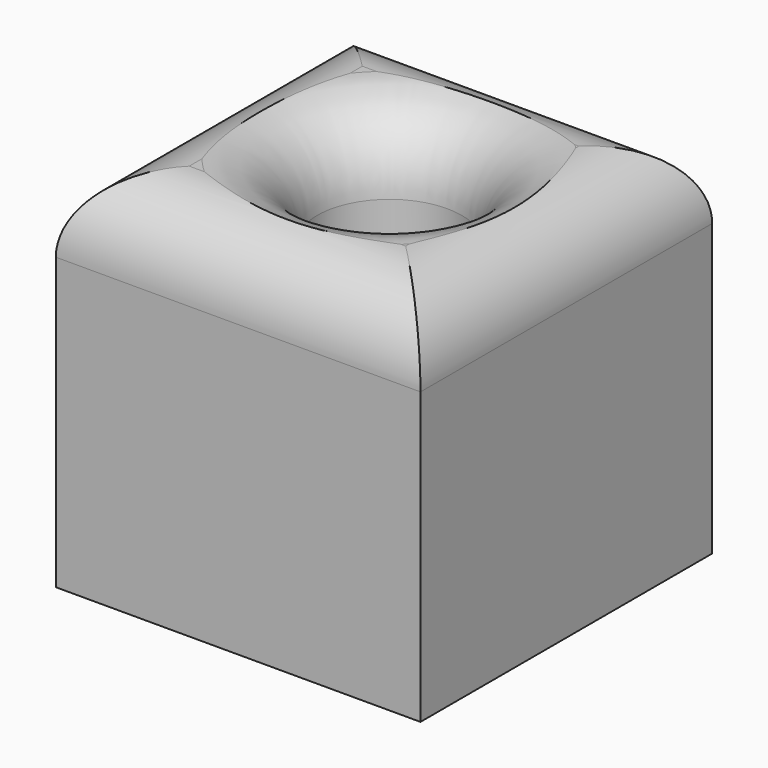
from build123d import *

# Parameters (mm, degrees)
F0_W        = 25
F0_H        = 25
F1_DEPTH    = 25
F2_R        = 4.9593089968
F3_DEPTH    = 25.4
F4_T1_DEPTH = 50.4
F4_T3_DEPTH = 50.4


# Not quite as in the source:
# - a fillet or chamfer that OpenCascade refuses, or shapes differently, is made with other operations: its cross-section is extruded or revolved along the edge and cut away or added


with BuildPart() as f1:
    # F0 (on Top) → F1 (new body)
    with BuildSketch(Plane.XY):
        with Locations((-12.5, -12.5)):
            Rectangle(F0_W, F0_H)
    extrude(amount=F1_DEPTH)

    # F2 (on face) → F3 (cut)
    with BuildSketch(Plane.XY.offset(25)):
        with Locations((-12.1455704793, -12.4741084874)):
            Circle(F2_R)
    extrude(amount=-F3_DEPTH, mode=Mode.SUBTRACT)

    # F4: fillet of radius 5.08 on 5 edges, made by hand

    # F4_s2 → F4_t1 (cut)
    with BuildSketch(Plane.XZ.offset(-12.7)):
        with BuildLine():
            ThreePointArc((0, 19.92), (-1.4878975516, 23.5121024484), (-5.08, 25))
            Line((-5.08, 25), (0, 25))
            Line((0, 25), (0, 19.92))
        make_face()
        with BuildLine():
            ThreePointArc((-19.92, 25), (-23.5121024484, 23.5121024484), (-25, 19.92))
            Line((-25, 19.92), (-25, 25))
            Line((-25, 25), (-19.92, 25))
        make_face()
    extrude(amount=F4_T1_DEPTH, mode=Mode.SUBTRACT)

    # F4_s4 → F4_t3 (cut)
    with BuildSketch(Plane.YZ.offset(-37.7)):
        with BuildLine():
            ThreePointArc((-25, 19.92), (-23.5121024484, 23.5121024484), (-19.92, 25))
            Line((-19.92, 25), (-25, 25))
            Line((-25, 25), (-25, 19.92))
        make_face()
        with BuildLine():
            ThreePointArc((0, 19.92), (-1.4878975516, 23.5121024484), (-5.08, 25))
            Line((-5.08, 25), (0, 25))
            Line((0, 25), (0, 19.92))
        make_face()
    extrude(amount=F4_T3_DEPTH, mode=Mode.SUBTRACT)

    # F4_s5 → F4_t6 (revolve, cut)
    with BuildSketch(Plane.XZ.offset(12.4741084874)):
        with BuildLine():
            ThreePointArc((-2.1062614826, 25), (-5.698363931, 23.5121024484), (-7.1862614826, 19.92))
            Line((-7.1862614826, 19.92), (-7.1862614826, 25))
            Line((-7.1862614826, 25), (-2.1062614826, 25))
        make_face()
    revolve(axis=Axis((-12.1455704793, -12.4741084874, 25), (0, 0, 1)), mode=Mode.SUBTRACT)


solid = f1.part
